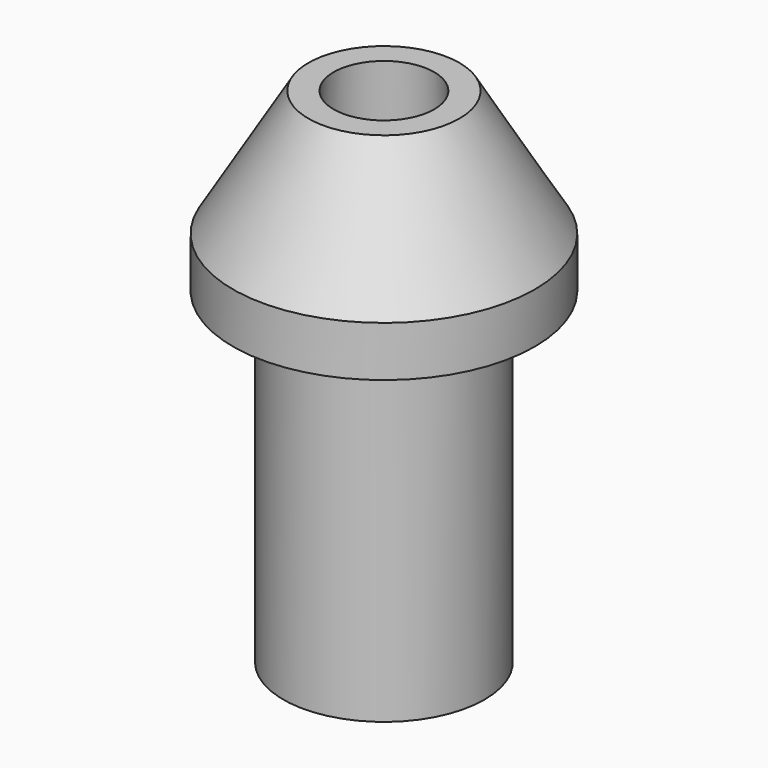
from build123d import *

# Parameters (mm, degrees)
F0_W = 2
F0_H = 2


# Not quite as in the source:
# - a feature names something its author has since deleted; it is built from what else it names


with BuildPart() as f1:
    # F0 (on Front) → F1 (revolve)
    with BuildSketch(Plane.XZ):
        with Locations((5, 14)):
            Rectangle(F0_W, F0_H)
        Polygon((4, 13), (4, 15), (3, 20), (2, 20), (3, 0), (4, 0), align=None)
        Polygon((3, 20), (4, 15), (6, 15), align=None)
    revolve(axis=Axis((0, 0, 10.5782048777), (0, 0, 1)))


solid = f1.part
